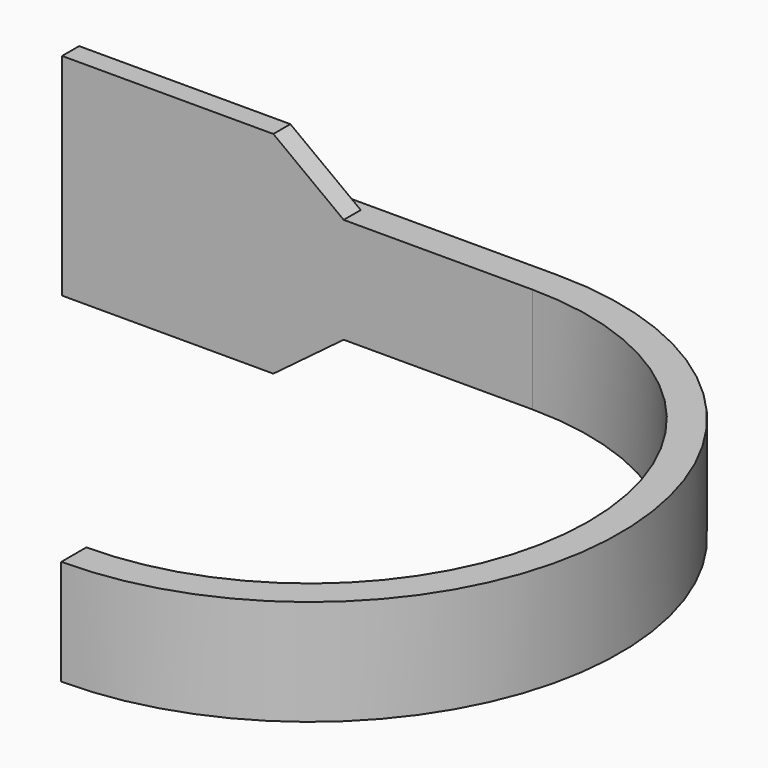
from build123d import *

# Parameters (mm, degrees)
F0_W     = 30.0332503393
F0_H     = 3.0297264457
F1_DEPTH = 15
F0_W_2   = 36.8763273582
F0_H_2   = 1.4379325638
F2_DEPTH = 7.5
F3_SIZE2 = 7.49999
F3_SIZE  = 9.99999
F4_SIZE2 = 7.49999
F4_SIZE  = 9.99999


# Not quite as in the source:
# - a fillet or chamfer is up to 0.001 mm smaller than in the source, because OpenCascade refuses the exact size


with BuildPart() as f1:
    # F0 (on Top) → F1 (new body, symmetric)
    with BuildSketch(Plane.XY):
        with Locations((-4.9947178923, 25.5465358496)):
            Rectangle(F0_W, F0_H)
    extrude(amount=F1_DEPTH, both=True)

    # F0 (on Top) → F2 (join, symmetric)
    with BuildSketch(Plane.XY):
        with Locations((-4.9947178923, 25.5465358496)):
            Rectangle(F0_W, F0_H)
        with Locations((28.4600709565, 27.7803653543)):
            Rectangle(F0_W_2, F0_H_2)
        with Locations((28.4600709565, 25.5465358496)):
            Rectangle(F0_W_2, F0_H)
        with BuildLine():
            ThreePointArc((46.8982346356, -58.3157722523), (89.586820298, -15.62718659), (46.8982346356, 27.0613990724))
            Line((46.8982346356, 27.0613990724), (46.8982346356, 24.0316726267))
            ThreePointArc((46.8982346356, 24.0316726267), (86.5570938523, -15.62718659), (46.8982346356, -55.2860458066))
            Line((46.8982346356, -55.2860458066), (46.8982346356, -58.3157722523))
        make_face()
        with BuildLine():
            Line((46.8982346356, 28.4993316362), (46.8982346356, 27.0613990724))
            ThreePointArc((46.8982346356, 27.0613990724), (89.586820298, -15.62718659), (46.8982346356, -58.3157722523))
            Line((46.8982346356, -58.3157722523), (46.8982346356, -59.7537048161))
            ThreePointArc((46.8982346356, -59.7537048161), (91.0247528617, -15.62718659), (46.8982346356, 28.4993316362))
        make_face()
    extrude(amount=F2_DEPTH, both=True)

    # F3 (size 10 and 7.5 in the source; OpenCascade refuses exactly that, so slightly less here)
    f3_edges = [f1.edges().sort_by_distance(p)[0] for p in [
        (10.021907, 25.546536, 7.5),
    ]]
    f3_side = f1.faces().sort_by_distance((11.219825, 27.780365, 7.5))[0]
    chamfer(f3_edges, length=F3_SIZE, length2=F3_SIZE2, reference=f3_side)

    # F4 (size 10 and 7.5 in the source; OpenCascade refuses exactly that, so slightly less here)
    f4_edges = [f1.edges().sort_by_distance(p)[0] for p in [
        (10.021907, 25.546536, -7.5),
    ]]
    f4_side = f1.faces().sort_by_distance((11.219825, 27.780365, -7.5))[0]
    chamfer(f4_edges, length=F4_SIZE, length2=F4_SIZE2, reference=f4_side)


solid = f1.part
